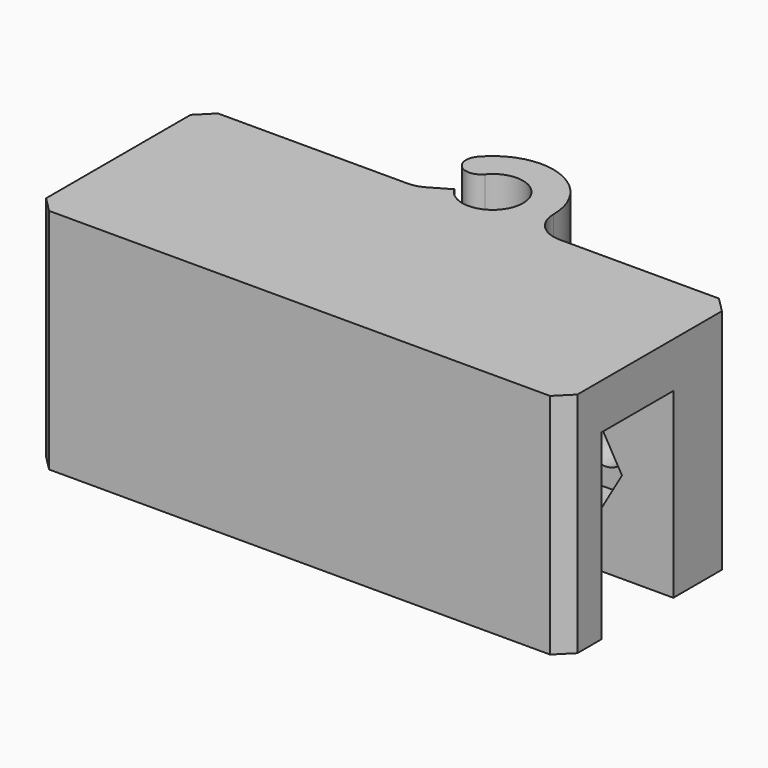
from build123d import *

# Parameters (mm, degrees)
F1_DEPTH = 17.5
F3_DEPTH = 15
F4_R     = 2
F5_SIZE  = 1
F7_DEPTH = 2.5
F8_R     = 1.5
F9_DEPTH = 2.5


with BuildPart() as f1:
    # F0 (on Right) → F1 (new body, symmetric)
    with BuildSketch(Plane.YZ):
        Polygon((-5, -15), (0, -15), (0, 0), (-13.9, 0), (-13.9, -15), (-10.9, -15), (-10.9, -3), (-5, -3), align=None)
    extrude(amount=F1_DEPTH, both=True)

    # F2 (on face) → F3 (join)
    with BuildSketch(Plane.XY):
        with BuildLine():
            Line((0, 0), (3.4641016151, 0))
            ThreePointArc((3.4641016151, 0), (2.2943057454, 5.2766081772), (-3.0641777725, 4.5711504387))
            ThreePointArc((-3.0641777725, 4.5711504387), (-2.940920939, 3.1623183859), (-1.5320888862, 3.2855752194))
            ThreePointArc((-1.5320888862, 3.2855752194), (1.8126155741, 2.8452365235), (0, 0))
        make_face()
        with BuildLine():
            Line((-3.4641016151, 0), (0, 0))
            ThreePointArc((0, 0), (-1, 0.2679491924), (-1.7320508076, 1))
            Line((-1.7320508076, 1), (-3.4641016151, 0))
        make_face()
    extrude(amount=-F3_DEPTH)

    # F4
    f4_edges = [f1.edges().sort_by_distance(p)[0] for p in [
        (3.464102, 0, -7.5),
        (-3.464102, 0, -7.5),
    ]]
    fillet(f4_edges, radius=F4_R)

    # F5
    f5_edges = [f1.edges().sort_by_distance(p)[0] for p in [
        (-17.5, 0, -7.5),
        (17.5, 0, -7.5),
        (-17.5, -13.9, -7.5),
        (17.5, -13.9, -7.5),
    ]]
    chamfer(f5_edges, length=F5_SIZE)

    # F6 (on face) → F7 (cut)
    with BuildSketch(Plane.XZ.offset(5)):
        Polygon((-12.5588457268, -11.7), (-9.4411542732, -11.7), (-7.8823085464, -9), (-9.4411542732, -6.3), (-12.5588457268, -6.3), (-14.1176914536, -9), align=None)
        Polygon((9.4411542732, -11.7), (12.5588457268, -11.7), (14.1176914536, -9), (12.5588457268, -6.3), (9.4411542732, -6.3), (7.8823085464, -9), align=None)
    extrude(amount=-F7_DEPTH, mode=Mode.SUBTRACT)

    # F8 (on face) → F9 (cut, through all)
    with BuildSketch(Plane(origin=(0, 0, 0), x_dir=(-1, 0, 0), z_dir=(0, 1, 0))):
        with Locations((-11, -9)):
            Circle(F8_R)
        with Locations((11, -9)):
            Circle(F8_R)
    extrude(amount=-F9_DEPTH, mode=Mode.SUBTRACT)


solid = f1.part
